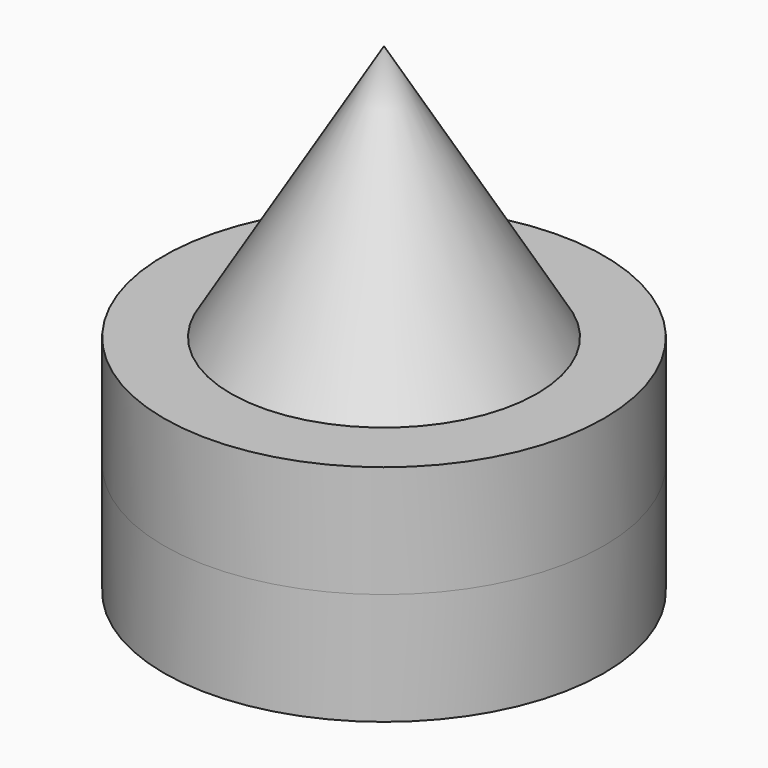
from build123d import *

# Parameters (mm, degrees)
F9_DEPTH = 14.224


# Not quite as in the source:
# - the program builds the solid bodies; features that only make, move or delete a surface that nothing else refers to are left out


with BuildPart() as f1:
    # F0 (on Front) → F1 (revolve)
    with BuildSketch(Plane.XZ):
        Polygon((0, 46.7339530587), (0, 0), (27.929758653, 0), align=None)
    revolve(axis=Axis((0, 0, 23.3669765294), (0, 0, 1)))

    # F9 (add, symmetric): a face of the model
    f9_faces = [f1.faces().sort_by_distance(p)[0] for p in [
        (0, 0, 0),
    ]]
    extrude(f9_faces, amount=F9_DEPTH, both=True)


solid = f1.part
